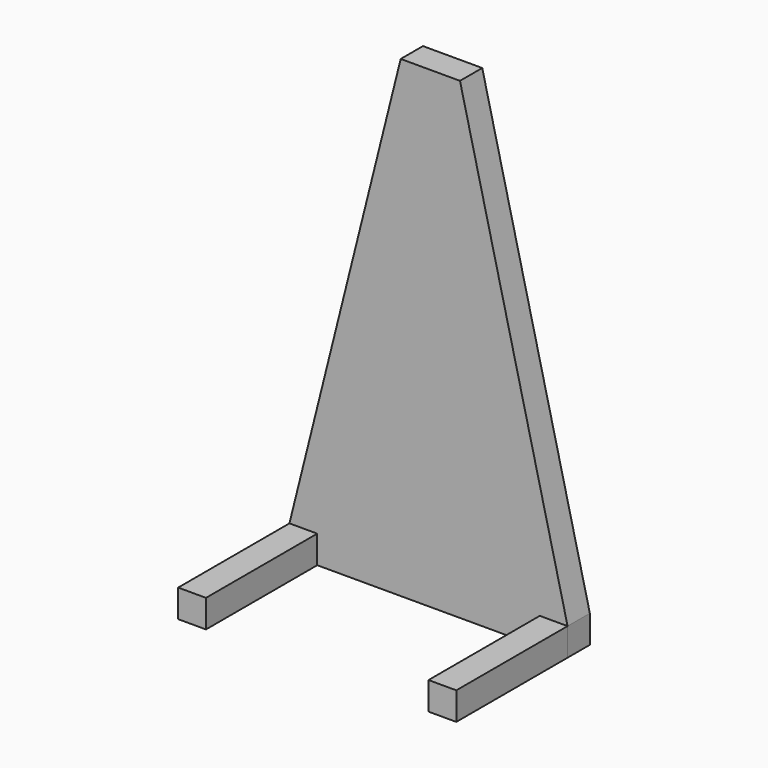
from build123d import *

# Parameters (mm, degrees)
F0_W      = 10
F0_H      = 50
F1_DEPTH  = 10
F4_DEPTH  = 10
F4_FACE_W = 100
F4_FACE_H = 10


with BuildPart() as f1:
    # F0 (on Top) → F1 (new body)
    with BuildSketch(Plane.XY):
        with Locations((-45, 0)):
            Rectangle(F0_W, F0_H)
    extrude(amount=F1_DEPTH)


with BuildPart() as f1b:
    # F0 (on Top) → F1, piece 2 (new body)
    with BuildSketch(Plane.XY):
        with Locations((45, 0)):
            Rectangle(F0_W, F0_H)
    extrude(amount=F1_DEPTH)


with BuildPart() as f4:
    # F0 (on Top) → F4 (new body)
    with BuildSketch(Plane.XY):
        Polygon((-40, 25), (40, 25), (50, 25), (50, 35), (-50, 35), (-50, 25), align=None)
    extrude(amount=F4_DEPTH)

    # F4_face (on face) → F5 section 0
    with BuildSketch(Plane(origin=(0, 30, 10), x_dir=(1, 0, 0), z_dir=(0, 0, 1))):
        Rectangle(F4_FACE_W, F4_FACE_H)
    # F3 (on offset) → F5 section 1
    with BuildSketch(Plane.XY.offset(170)):
        Polygon((0, 35), (-10, 35), (-10, 25), (11.3194556907, 25), (11.3194556907, 35), align=None)
    loft()


solid = Compound([f1.part, f1b.part, f4.part])
